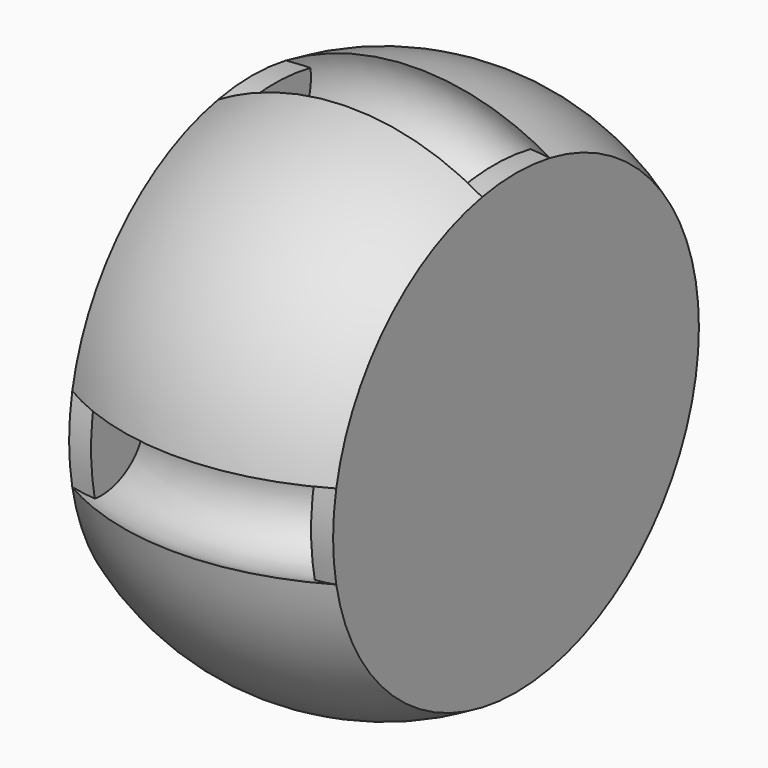
from build123d import *

# Parameters (mm, degrees)
F2_R     = 5.25
F4_R     = 25.9807621135
F5_DEPTH = 2.5


# Not quite as in the source:
# - a pattern or mirror of a feature is missing from the dataset's text; its kind, count and spacing are read off the source's solid


with BuildPart() as f1:
    # F0 (on Front) → F1 (revolve)
    with BuildSketch(Plane.XZ):
        with BuildLine():
            Line((-15, 25.9807621135), (-15, 0))
            Line((-15, 0), (15, 0))
            Line((15, 0), (15, 25.9807621135))
            ThreePointArc((15, 25.9807621135), (0, 30), (-15, 25.9807621135))
        make_face()
    revolve(axis=Axis((0, 0, 0), (1, 0, 0)))

    # F2 (on Right) → F3 (revolve, cut)
    with BuildSketch(Plane.YZ):
        with Locations((0, -27.5)):
            Circle(F2_R)
    f3 = revolve(axis=Axis((0, 15, 0), (0, 1, 0)), mode=Mode.SUBTRACT)

    # F3_copies: F3 across plane
    add(f3.mirror(Plane(origin=(0, -1e-06, -1e-06), x_dir=(0, -0.7071084838, 0.7071050786), z_dir=(0, -0.7071050786, -0.7071084838))), mode=Mode.SUBTRACT)

    # F4 (on face) → F5 (join)
    with BuildSketch(Plane(origin=(-15, 0, 0), x_dir=(0, -1, 0), z_dir=(-1, 0, 0))):
        Circle(F4_R)
    extrude(amount=-F5_DEPTH)

    # F6: F1 across plane


with BuildPart() as f1_1:
    add(f1.part)
    add(f1.part.mirror(Plane.YZ))


solid = f1_1.part
